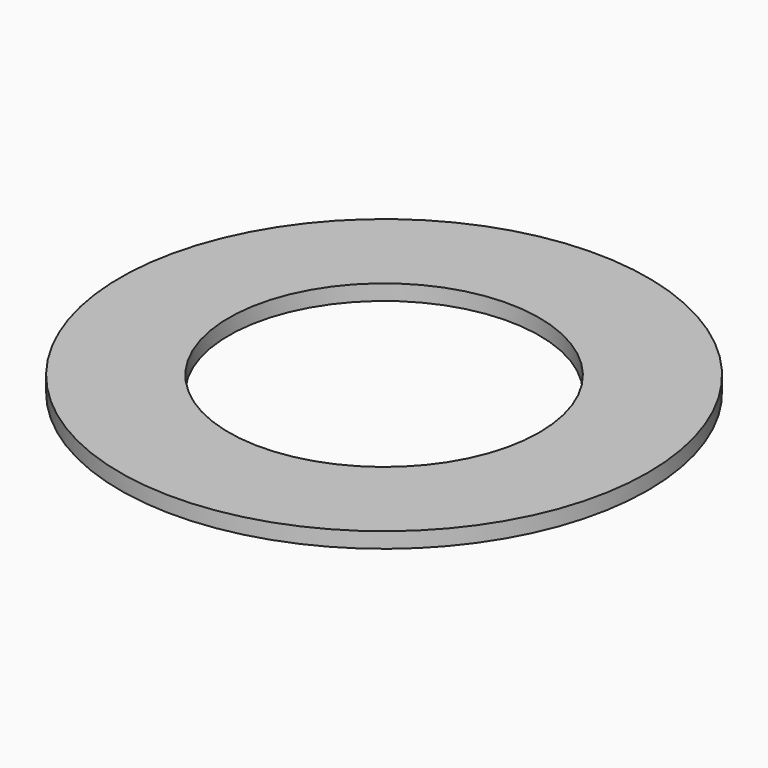
from build123d import *

# Parameters (mm, degrees)
F0_R     = 17
F0_R_2   = 16.2
F1_DEPTH = 1
F3_R     = 10
F4_DEPTH = 3


# Not quite as in the source:
# - a feature names something its author has since deleted; it is built from what else it names
# - the program builds the solid bodies; features that only make, move or delete a surface that nothing else refers to are left out


with BuildPart() as f1:
    # F0 (on Top) → F1 (new body)
    with BuildSketch(Plane.XY):
        Circle(F0_R)
        Circle(F0_R_2, mode=Mode.SUBTRACT)
        Circle(F0_R_2)
    extrude(amount=F1_DEPTH)

    # F3 (on face) → F4 (cut)
    with BuildSketch(Plane(origin=(0, 0, 0), x_dir=(1, 0, 0), z_dir=(0, 0, -1))):
        Circle(F3_R)
    extrude(amount=-F4_DEPTH, mode=Mode.SUBTRACT)


solid = f1.part
